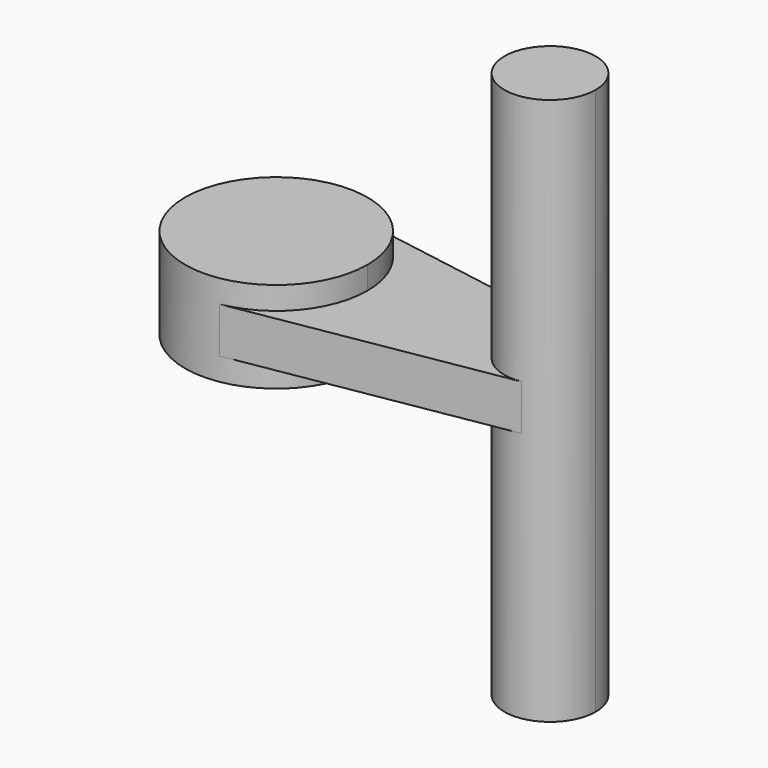
from build123d import *

# Parameters (mm, degrees)
F1_DEPTH = 12.7
F2_DEPTH = 6.35
F3_DEPTH = 76.2


# Not quite as in the source:
# - the program builds the solid bodies; features that only make, move or delete a surface that nothing else refers to are left out


with BuildPart() as f1:
    # F0 (on Top) → F1 (new body, symmetric)
    with BuildSketch(Plane.XY):
        with BuildLine():
            ThreePointArc((4.2333333333, -25.0447377485), (19.399570442, -16.3956294989), (25.4, 0))
            ThreePointArc((25.4, 0), (19.399570442, 16.3956294989), (4.2333333333, 25.0447377485))
            ThreePointArc((4.2333333333, 25.0447377485), (-25.4, 0), (4.2333333333, -25.0447377485))
        make_face()
    extrude(amount=F1_DEPTH, both=True)

    # F0 (on Top) → F2 (join, symmetric)
    with BuildSketch(Plane.XY):
        with BuildLine():
            ThreePointArc((4.2333333333, 25.0447377485), (19.399570442, 16.3956294989), (25.4, 0))
            ThreePointArc((25.4, 0), (19.399570442, -16.3956294989), (4.2333333333, -25.0447377485))
            Line((4.2333333333, -25.0447377485), (78.3166666667, -12.5223688742))
            ThreePointArc((78.3166666667, -12.5223688742), (63.5, 0), (78.3166666667, 12.5223688742))
            Line((78.3166666667, 12.5223688742), (4.2333333333, 25.0447377485))
        make_face()
    extrude(amount=F2_DEPTH, both=True)


with BuildPart() as f3:
    # F0 (on Top) → F3 (new body, symmetric)
    with BuildSketch(Plane.XY):
        with BuildLine():
            ThreePointArc((88.9, 0), (85.899785221, 8.1978147495), (78.3166666667, 12.5223688742))
            ThreePointArc((78.3166666667, 12.5223688742), (63.5, 0), (78.3166666667, -12.5223688742))
            ThreePointArc((78.3166666667, -12.5223688742), (85.899785221, -8.1978147495), (88.9, 0))
        make_face()
    extrude(amount=F3_DEPTH, both=True)


solid = Compound([f1.part, f3.part])
